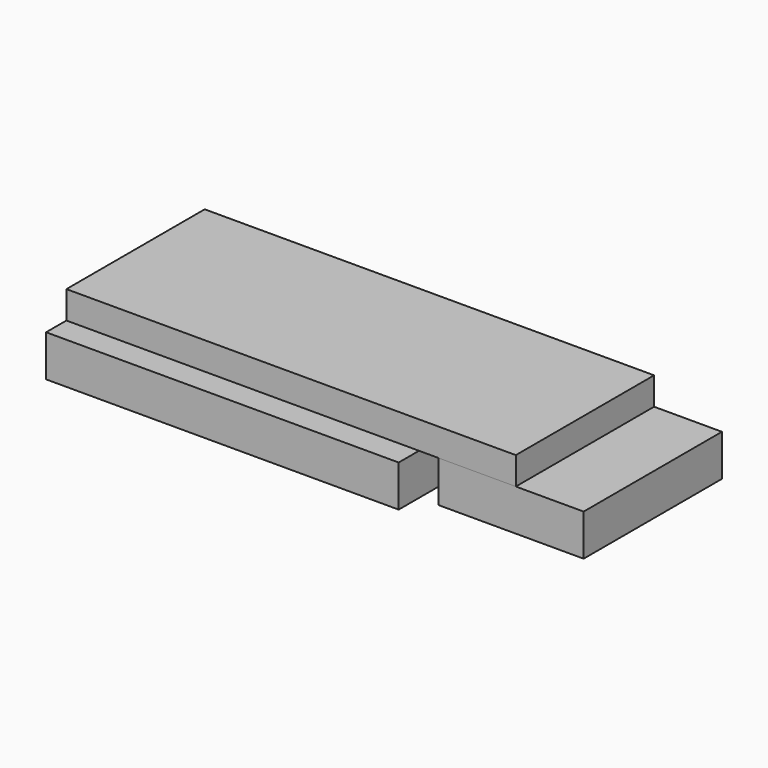
from build123d import *

# Parameters (mm, degrees)
F0_W     = 51
F0_H     = 33.5
F1_DEPTH = 6
F2_W     = 65
F2_H     = 25
F3_DEPTH = 4
F4_W     = 21
F4_H     = 25
F5_DEPTH = 6


# Not quite as in the source:
# - a feature names something its author has since deleted; it is built from what else it names


with BuildPart() as f1:
    # F0 (on Top) → F1 (new body)
    with BuildSketch(Plane.XY):
        with Locations((25.5, 16.75)):
            Rectangle(F0_W, F0_H)
    extrude(amount=F1_DEPTH)


with BuildPart() as f3:
    # F2 (on face) → F3 (new body)
    with BuildSketch(Plane.XY.offset(6)):
        with Locations((32.5, 16.1751881707)):
            Rectangle(F2_W, F2_H)
    extrude(amount=F3_DEPTH)


with BuildPart() as f5:
    # F4 (on face) → F5 (new body)
    with BuildSketch(Plane(origin=(0, 0, 6), x_dir=(1, 0, 0), z_dir=(0, 0, -1))):
        with Locations((64.3100422634, -16.1751881707)):
            Rectangle(F4_W, F4_H)
    extrude(amount=F5_DEPTH)


solid = Compound([f1.part, f3.part, f5.part])
